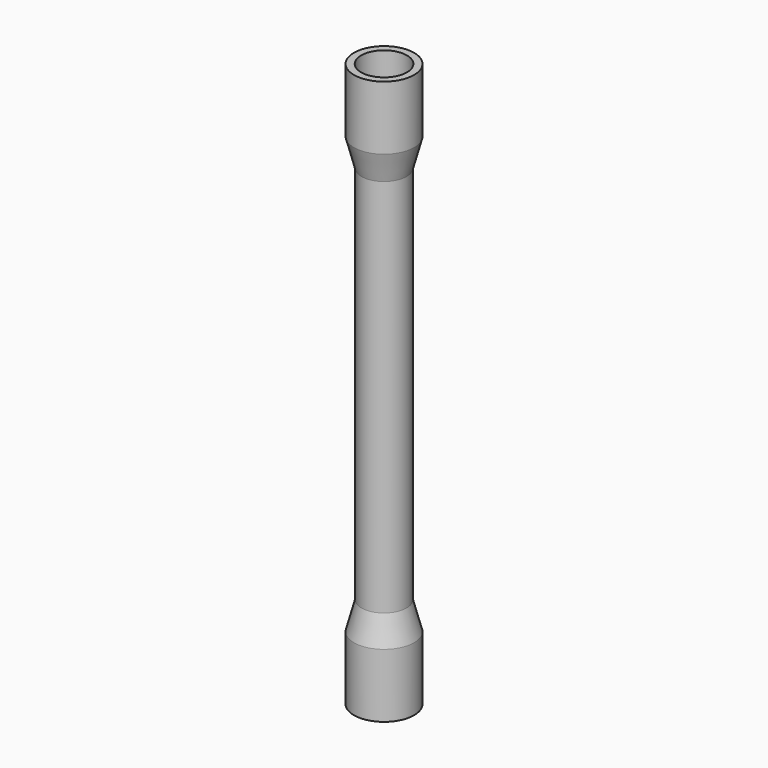
from build123d import *

# Parameters (mm, degrees)
F0_R          = 6
F1_DEPTH      = 50
F1_DEPTH_BACK = 50
F2_R          = 8
F2_R_2        = 6
F4_DEPTH      = 25
F3_R          = 8
F3_R_2        = 6
F5_DEPTH      = 25
F6_S5_R       = 6
F6_T6_DEPTH   = 14
F6_S11_R      = 6
F6_T12_DEPTH  = 14
F7_R          = 6.1
F8_DEPTH      = 9
F9_R          = 6.1
F10_DEPTH     = 9


# Not quite as in the source:
# - a fillet or chamfer that OpenCascade refuses, or shapes differently, is made with other operations: its cross-section is extruded or revolved along the edge and cut away or added


with BuildPart() as f1:
    # F0 (on Top) → F1 (new body, two sides)
    with BuildSketch(Plane.XY) as f1_sk:
        Circle(F0_R)
    extrude(amount=F1_DEPTH)
    extrude(f1_sk.sketch, amount=-F1_DEPTH_BACK)

    # F2 (on face) → F4 (join)
    with BuildSketch(Plane.XY.offset(50)):
        Circle(F2_R)
        Circle(F2_R_2, mode=Mode.SUBTRACT)
        Circle(F2_R_2)
    extrude(amount=F4_DEPTH)

    # F3 (on face) → F5 (join)
    with BuildSketch(Plane(origin=(0, 0, -50), x_dir=(1, 0, 0), z_dir=(0, 0, -1))):
        Circle(F3_R)
        Circle(F3_R_2, mode=Mode.SUBTRACT)
        Circle(F3_R_2)
    extrude(amount=F5_DEPTH)

    # F6: chamfer of 8 x 2.1435935394 on 2 edges, made by hand


with BuildPart() as f6_tool2:
    # F6_s3 → F6_t4 (revolve)
    with BuildSketch(Plane.XZ):
        Polygon((8, -58), (5.8564064606, -50), (8, -50), align=None)
    revolve(axis=Axis((0, 0, -50), (0, 0, -1)))

    # F6_s5 → F6_t6 (cut, symmetric)
    with BuildSketch(Plane.XY.offset(-54)):
        Circle(F6_S5_R)
    extrude(amount=F6_T6_DEPTH, both=True, mode=Mode.SUBTRACT)


with BuildPart() as f1_1:
    add(f1.part)

    # F6_t1: cut F6_tool2
    add(f6_tool2.part, mode=Mode.SUBTRACT)


with BuildPart() as f6_tool8:
    # F6_s9 → F6_t10 (revolve)
    with BuildSketch(Plane.XZ):
        Polygon((5.8564064606, 50), (8, 58), (8, 50), align=None)
    revolve(axis=Axis((0, 0, 50), (0, 0, 1)))

    # F6_s11 → F6_t12 (cut, symmetric)
    with BuildSketch(Plane.XY.offset(54)):
        Circle(F6_S11_R)
    extrude(amount=F6_T12_DEPTH, both=True, mode=Mode.SUBTRACT)


with BuildPart() as f1_2:
    add(f1_1.part)

    # F6_t7: cut F6_tool8
    add(f6_tool8.part, mode=Mode.SUBTRACT)

    # F7 (on face) → F8 (cut)
    with BuildSketch(Plane(origin=(0, 0, -75), x_dir=(1, 0, 0), z_dir=(0, 0, -1))):
        Circle(F7_R)
    extrude(amount=-F8_DEPTH, mode=Mode.SUBTRACT)

    # F9 (on face) → F10 (cut)
    with BuildSketch(Plane.XY.offset(75)):
        Circle(F9_R)
    extrude(amount=-F10_DEPTH, mode=Mode.SUBTRACT)


solid = f1_2.part
